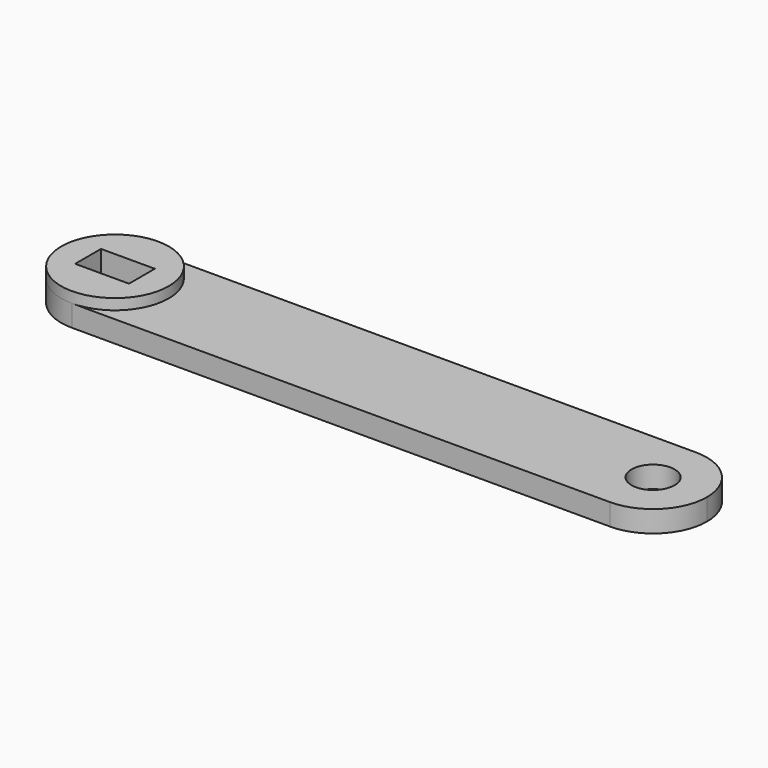
from build123d import *

# Parameters (mm, degrees)
F0_W          = 60
F0_H          = 10
F1_DEPTH      = 2
F2_R          = 4.99999
F3_R          = 5
F4_DEPTH      = 1
F5_W          = 5
F5_H          = 3
F6_DEPTH      = 1.001
F6_DEPTH_BACK = 2.001
F7_R          = 2
F8_DEPTH      = 2.001


# Not quite as in the source:
# - a fillet or chamfer is up to 0.001 mm smaller than in the source, because OpenCascade refuses the exact size


with BuildPart() as f1:
    # F0 (on Top) → F1 (new body)
    with BuildSketch(Plane.XY):
        with Locations((30, -5)):
            Rectangle(F0_W, F0_H)
    extrude(amount=F1_DEPTH)

    # F2 (radius 5 in the source; OpenCascade refuses exactly that, so slightly less here)
    f2_edges = [f1.edges().sort_by_distance(p)[0] for p in [
        (0, -10, 1),
        (0, 0, 1),
        (60, -10, 1),
        (60, 0, 1),
    ]]
    fillet(f2_edges, radius=F2_R)

    # F3 (on face) → F4 (join)
    with BuildSketch(Plane.XY.offset(2)):
        with Locations((5, -5)):
            Circle(F3_R)
    extrude(amount=F4_DEPTH)

    # F5 (on face) → F6 (cut, two sides)
    with BuildSketch(Plane.XY.offset(2)) as f6_sk:
        with Locations((5, -5)):
            Rectangle(F5_W, F5_H)
    extrude(amount=F6_DEPTH, mode=Mode.SUBTRACT)
    extrude(f6_sk.sketch, amount=-F6_DEPTH_BACK, mode=Mode.SUBTRACT)

    # F7 (on face) → F8 (cut, through all)
    with BuildSketch(Plane.XY.offset(2)):
        with Locations((55, -5)):
            Circle(F7_R)
    extrude(amount=-F8_DEPTH, mode=Mode.SUBTRACT)


solid = f1.part
